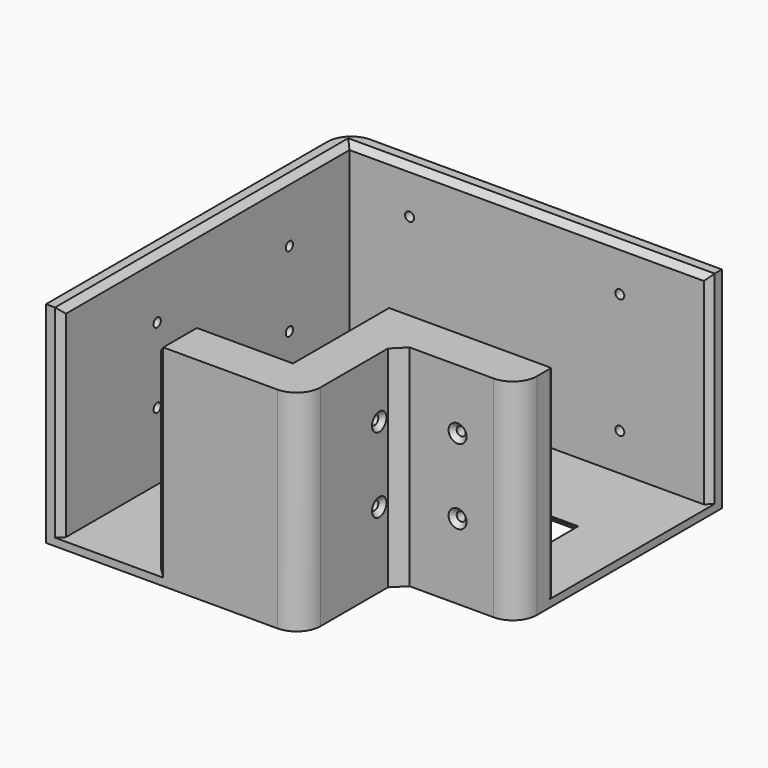
from build123d import *

# Parameters (mm, degrees)
F1_DEPTH        = 3.175
F2_DEPTH        = 88.9
F4_D            = 3.81
F4_DEPTH        = 25.4
F4_CSINK_D      = 7.62
F4_CSINK_ANGLE  = 90
F4_TIP          = 1.1446394792
F6_D            = 3.81
F6_DEPTH        = 25.4
F6_CSINK_D      = 7.62
F6_CSINK_ANGLE  = 90
F6_TIP          = 1.1446394792
F8_D            = 3.81
F8_DEPTH        = 25.4
F8_CSINK_D      = 7.62
F8_CSINK_ANGLE  = 90
F8_TIP          = 1.1446394792
F10_D           = 3.81
F10_DEPTH       = 25.4
F10_CSINK_D     = 7.62
F10_CSINK_ANGLE = 90
F10_TIP         = 1.1446394792
F11_T1_DEPTH    = 88.9
F11_T3_DEPTH    = 6.4524666085
F11_T5_DEPTH    = 6.4524666085
F11_T7_DEPTH    = 98.7891495789
F11_T9_DEPTH    = 115.0282991577
F11_T11_DEPTH   = 53.7041495789
F11_T13_DEPTH   = 63.8641495789
F11_T15_DEPTH   = 99.7882991577
F11_T17_DEPTH   = 48.9882991577
F11_T23_DEPTH   = 63.8641495789
F11_T27_DEPTH   = 53.7041495789
F12_R           = 10.16
F13_T1_DEPTH    = 91.44
F13_T3_DEPTH    = 52.2520747895
F13_T5_DEPTH    = 40.64
F13_T7_DEPTH    = 158.9320747894
F13_T9_DEPTH    = 158.9320747894
F13_T11_DEPTH   = 88.591569985
F13_T13_DEPTH   = 92.2570747894
F13_T15_DEPTH   = 49.9301865966
F13_T17_DEPTH   = 40.64
F13_T19_DEPTH   = 89.1181118071
F13_T25_DEPTH   = 47.1720747894
F13_T29_DEPTH   = 97.9720747894
F13_T36_DEPTH   = 95.6501865965
F13_T40_DEPTH   = 97.9720747894
F13_T47_DEPTH   = 47.1720747894
F13_T51_DEPTH   = 58.7841495789
F13_T58_DEPTH   = 158.9320747894
F13_S59_R       = 10.16
F13_T60_DEPTH   = 81
F13_T64_DEPTH   = 158.9320747894
F13_S66_R       = 10.16
F13_T67_DEPTH   = 81
F13_T73_DEPTH   = 56.462261386
F13_T77_DEPTH   = 47.1720747894
F13_T84_DEPTH   = 47.1720747894
F13_T88_DEPTH   = 95.6501865965


# Not quite as in the source:
# - a fillet or chamfer that OpenCascade refuses, or shapes differently, is made with other operations: its cross-section is extruded or revolved along the edge and cut away or added
# - a feature of the source that left no trace in its solid (it failed there, or was rolled back) is left out
# - a feature names something its author has since deleted; it is built from what else it names


with BuildPart() as f1:
    # F0 (on Top) → F1 (new body)
    with BuildSketch(Plane.XY):
        Polygon((-206.9763107598, 19.3472499192), (-359.3763107598, 19.3472499192), (-359.3763107598, -133.0527500808), (-321.2763107598, -133.0527500808), (-321.2763107598, -110.1927500808), (-321.2763107598, -18.7527500808), (-232.3763107598, -18.7527500808), (-232.1581989527, -18.7527500808), (-232.1581989527, -59.3927500808), (-206.9763107598, -59.3927500808), align=None)
    extrude(amount=F1_DEPTH)

    # F0 (on Top) → F2 (join)
    with BuildSketch(Plane.XY):
        Polygon((-206.9763107598, -82.2527500808), (-206.9763107598, -59.3927500808), (-232.1581989527, -59.3927500808), (-232.3763107598, -59.3927500808), (-280.6363107598, -59.3927500808), (-280.6363107598, -110.1927500808), (-321.2763107598, -110.1927500808), (-321.2763107598, -133.0527500808), (-257.7763107598, -133.0527500808), (-257.7763107598, -82.2527500808), align=None)
        Polygon((-359.3763107598, -133.0527500808), (-359.3763107598, 19.3472499192), (-206.9763107598, 19.3472499192), (-206.9763107598, 25.6972499192), (-365.7263107598, 25.6972499192), (-365.7263107598, -133.0527500808), align=None)
    extrude(amount=F2_DEPTH)

    # F4
    with Locations(Plane.XZ.offset(82.2527500808)):
        with Locations((-232.3763107598, 63.5), (-232.3763107598, 31.75)):
            CounterSinkHole(F4_D / 2, F4_CSINK_D / 2, depth=F4_DEPTH, counter_sink_angle=F4_CSINK_ANGLE)
            with Locations((0, 0, -(F4_DEPTH + F4_TIP / 2))):  # 118° drill point
                Cone(0, F4_D / 2, F4_TIP, mode=Mode.SUBTRACT)

    # F6
    with Locations(Plane.YZ.offset(-257.7763107598)):
        with Locations((-91.9047519565, 63.5), (-91.9047519565, 31.75)):
            CounterSinkHole(F6_D / 2, F6_CSINK_D / 2, depth=F6_DEPTH, counter_sink_angle=F6_CSINK_ANGLE)
            with Locations((0, 0, -(F6_DEPTH + F6_TIP / 2))):  # 118° drill point
                Cone(0, F6_D / 2, F6_TIP, mode=Mode.SUBTRACT)

    # F8
    with Locations(Plane(origin=(-365.7263107598, 0, 0), x_dir=(0, -1, 0), z_dir=(-1, 0, 0))):
        with Locations((12.4027500808, 63.5), (82.2527500808, 63.5), (82.2527500808, 31.75), (12.4027500808, 31.75)):
            CounterSinkHole(F8_D / 2, F8_CSINK_D / 2, depth=F8_DEPTH, counter_sink_angle=F8_CSINK_ANGLE)
            with Locations((0, 0, -(F8_DEPTH + F8_TIP / 2))):  # 118° drill point
                Cone(0, F8_D / 2, F8_TIP, mode=Mode.SUBTRACT)

    # F10
    with Locations(Plane(origin=(0, 25.6972499192, 0), x_dir=(-1, 0, 0), z_dir=(0, 1, 0))):
        with Locations((245.0763107598, 69.85), (245.0763107598, 19.05), (333.9763107598, 19.05), (333.9763107598, 69.85)):
            CounterSinkHole(F10_D / 2, F10_CSINK_D / 2, depth=F10_DEPTH, counter_sink_angle=F10_CSINK_ANGLE)
            with Locations((0, 0, -(F10_DEPTH + F10_TIP / 2))):  # 118° drill point
                Cone(0, F10_D / 2, F10_TIP, mode=Mode.SUBTRACT)

    # F11: chamfer of 5.08 on 10 edges, made by hand

    # F11_s2 → F11_t1 (join)
    with BuildSketch(Plane.XY):
        Polygon((-252.6963107598, -82.2527500808), (-257.7763107598, -87.3327500808), (-257.7763107598, -82.2527500808), align=None)
    extrude(amount=F11_T1_DEPTH)

    # F11_s4 → F11_t3 (cut)
    with BuildSketch(Plane(origin=(-96.6078535597, 96.6078535597, 96.6078535597), x_dir=(-0.7071067812, -0.7071067812, 0), z_dir=(-0.5773502692, 0.5773502692, 0.5773502692))):
        Polygon((301.5025963442, -15.6618580633), (305.0946987926, -9.4401541166), (308.686801241, -15.6618580633), align=None)
    extrude(amount=F11_T3_DEPTH, mode=Mode.SUBTRACT)

    # F11_s6 → F11_t5 (cut)
    with BuildSketch(Plane(origin=(-99.9945202263, 99.9945202263, 99.9945202263), x_dir=(-0.7071067812, -0.7071067812, 0), z_dir=(-0.5773502692, 0.5773502692, 0.5773502692))):
        Polygon((240.4368547209, -13.5879567477), (236.8447522725, -19.8096606944), (244.0289571693, -19.8096606944), align=None)
    extrude(amount=F11_T5_DEPTH, mode=Mode.SUBTRACT)

    # F11_s8 → F11_t7 (cut)
    with BuildSketch(Plane.XY.offset(3.175)):
        Polygon((-316.1963107598, -110.1927500808), (-321.2763107598, -115.2727500808), (-321.2763107598, -110.1927500808), align=None)
        Polygon((-316.1963107598, -133.0527500808), (-321.2763107598, -127.9727500808), (-321.2763107598, -133.0527500808), align=None)
        Polygon((-206.9763107598, -64.4727500808), (-212.0563107598, -59.3927500808), (-206.9763107598, -59.3927500808), align=None)
    extrude(amount=F11_T7_DEPTH, mode=Mode.SUBTRACT)

    # F11_s10 → F11_t9 (cut)
    with BuildSketch(Plane.XY.offset(-13.0641495789)):
        Polygon((-275.5563107598, -59.3927500808), (-280.6363107598, -64.4727500808), (-280.6363107598, -59.3927500808), align=None)
    extrude(amount=F11_T9_DEPTH, mode=Mode.SUBTRACT)

    # F11_s12 → F11_t11 (cut)
    with BuildSketch(Plane.YZ.offset(-334.3404603386)):
        Polygon((-115.2727500808, 88.9), (-110.1927500808, 83.82), (-110.1927500808, 88.9), align=None)
    extrude(amount=F11_T11_DEPTH, mode=Mode.SUBTRACT)

    # F11_s14 → F11_t13 (cut)
    with BuildSketch(Plane.XZ.offset(46.328600502)):
        Polygon((-275.5563107598, 88.9), (-280.6363107598, 83.82), (-280.6363107598, 88.9), align=None)
    extrude(amount=F11_T13_DEPTH, mode=Mode.SUBTRACT)

    # F11_s16 → F11_t15 (cut)
    with BuildSketch(Plane.YZ.offset(-293.7004603386)):
        Polygon((-64.4727500808, 88.9), (-59.3927500808, 83.82), (-59.3927500808, 88.9), align=None)
    extrude(amount=F11_T15_DEPTH, mode=Mode.SUBTRACT)

    # F11_s18 → F11_t17 (cut)
    with BuildSketch(Plane.XZ.offset(97.128600502)):
        Polygon((-316.1963107598, 88.9), (-321.2763107598, 83.82), (-321.2763107598, 88.9), align=None)
    extrude(amount=F11_T17_DEPTH, mode=Mode.SUBTRACT)


with BuildPart() as f11_tool21:
    # F11_s22 → F11_t23 (new body)
    with BuildSketch(Plane.XZ.offset(59.3927500808)):
        Polygon((-275.5563107598, 88.9), (-280.6363107598, 83.82), (-280.6363107598, 88.9), align=None)
    extrude(amount=F11_T23_DEPTH)

    split(bisect_by=Plane.XZ.offset(110.1927500808), keep=Keep.TOP)


with BuildPart() as f11_tool25:
    # F11_s26 → F11_t27 (new body)
    with BuildSketch(Plane.YZ.offset(-267.5721611809)):
        Polygon((-115.2727500808, 88.9), (-110.1927500808, 83.82), (-110.1927500808, 88.9), align=None)
    extrude(amount=-F11_T27_DEPTH)

    split(bisect_by=Plane.YZ.offset(-280.6363107598), keep=Keep.TOP)


with BuildPart() as f11_tool21_1:
    add(f11_tool21.part)

    # F11_t29: intersect F11_tool25
    add(f11_tool25.part, mode=Mode.INTERSECT)


with BuildPart() as f1_1:
    add(f1.part)

    # F11_t19: cut F11_tool21
    add(f11_tool21_1.part, mode=Mode.SUBTRACT)

    # F12
    f12_edges = [f1_1.edges().sort_by_distance(p)[0] for p in [
        (-257.776311, -133.05275, 44.45),
        (-206.976311, -82.25275, 44.45),
        (-365.726311, 25.69725, 44.45),
    ]]
    fillet(f12_edges, radius=F12_R)

    # F13: chamfer of 2.54 on 11 edges, made by hand

    # F13_s2 → F13_t1 (cut)
    with BuildSketch(Plane.XZ.offset(18.7527500808)):
        Polygon((-323.8163107598, 0), (-321.2763107598, 2.54), (-321.2763107598, 0), align=None)
    extrude(amount=F13_T1_DEPTH, mode=Mode.SUBTRACT)

    # F13_s4 → F13_t3 (cut)
    with BuildSketch(Plane.XZ.offset(57.9406752914)):
        Polygon((-278.0963107598, 0), (-280.6363107598, 2.54), (-280.6363107598, 0), align=None)
    extrude(amount=F13_T3_DEPTH, mode=Mode.SUBTRACT)

    # F13_s6 → F13_t5 (cut)
    with BuildSketch(Plane.YZ.offset(-321.2763107598)):
        Polygon((-112.7327500808, 0), (-110.1927500808, 2.54), (-110.1927500808, 0), align=None)
    extrude(amount=F13_T5_DEPTH, mode=Mode.SUBTRACT)

    # F13_s8 → F13_t7 (cut)
    with BuildSketch(Plane.YZ.offset(-359.3763107598)):
        Polygon((21.8872499192, 88.9), (19.3472499192, 86.36), (19.3472499192, 88.9), align=None)
    extrude(amount=F13_T7_DEPTH, mode=Mode.SUBTRACT)

    # F13_s10 → F13_t9 (cut)
    with BuildSketch(Plane.XZ.offset(-19.3472499192)):
        Polygon((-361.9163107598, 88.9), (-359.3763107598, 86.36), (-359.3763107598, 88.9), align=None)
    extrude(amount=F13_T9_DEPTH, mode=Mode.SUBTRACT)

    # F13_s12 → F13_t11 (cut)
    with BuildSketch(Plane.XY.offset(3.175)):
        Polygon((-206.9763107598, -65.5248525292), (-207.7202595356, -63.728801305), (-206.9763107598, -64.4727500808), align=None)
    extrude(amount=F13_T11_DEPTH, mode=Mode.SUBTRACT)

    # F13_s14 → F13_t13 (cut)
    with BuildSketch(Plane.XY.offset(3.175)):
        Polygon((-206.9763107598, 21.8872499192), (-209.5163107598, 19.3472499192), (-206.9763107598, 19.3472499192), align=None)
        Polygon((-361.9163107598, -133.0527500808), (-359.3763107598, -130.5127500808), (-359.3763107598, -133.0527500808), align=None)
    extrude(amount=F13_T13_DEPTH, mode=Mode.SUBTRACT)

    # F13_s16 → F13_t15 (cut)
    with BuildSketch(Plane.YZ.offset(-282.0883855492)):
        Polygon((-61.9327500808, 0), (-59.3927500808, 2.54), (-59.3927500808, 0), align=None)
    extrude(amount=F13_T15_DEPTH, mode=Mode.SUBTRACT)

    # F13_s18 → F13_t17 (cut)
    with BuildSketch(Plane.XZ.offset(18.7527500808)):
        Polygon((-229.6181989527, 0), (-232.1581989527, 2.54), (-232.1581989527, 0), align=None)
    extrude(amount=F13_T17_DEPTH, mode=Mode.SUBTRACT)

    # F13_s20 → F13_t19 (cut)
    with BuildSketch(Plane.YZ.offset(-321.2763107598)):
        Polygon((-16.2127500808, 0), (-18.7527500808, 2.54), (-18.7527500808, 0), align=None)
    extrude(amount=F13_T19_DEPTH, mode=Mode.SUBTRACT)


with BuildPart() as f13_tool23:
    # F13_s24 → F13_t25 (new body)
    with BuildSketch(Plane.YZ.offset(-280.6363107598)):
        Polygon((-112.7327500808, 0), (-110.1927500808, 2.54), (-110.1927500808, 0), align=None)
    extrude(amount=-F13_T25_DEPTH)

    split(bisect_by=Plane.YZ.offset(-321.2763107598), keep=Keep.BOTTOM)


with BuildPart() as f13_tool27:
    # F13_s28 → F13_t29 (new body)
    with BuildSketch(Plane.XZ.offset(116.7248248703)):
        Polygon((-323.8163107598, 0), (-321.2763107598, 2.54), (-321.2763107598, 0), align=None)
    extrude(amount=-F13_T29_DEPTH)

    split(bisect_by=Plane.XZ.offset(110.1927500808), keep=Keep.TOP)


with BuildPart() as f13_tool23_1:
    add(f13_tool23.part)

    # F13_t31: intersect F13_tool27
    add(f13_tool27.part, mode=Mode.INTERSECT)


with BuildPart() as f1_2:
    add(f1_1.part)

    # F13_t21: cut F13_tool23
    add(f13_tool23_1.part, mode=Mode.SUBTRACT)


with BuildPart() as f13_tool34:
    # F13_s35 → F13_t36 (new body)
    with BuildSketch(Plane.YZ.offset(-327.8083855492)):
        Polygon((-16.2127500808, 0), (-18.7527500808, 2.54), (-18.7527500808, 0), align=None)
    extrude(amount=F13_T36_DEPTH)

    split(bisect_by=Plane.YZ.offset(-321.2763107598), keep=Keep.BOTTOM)


with BuildPart() as f13_tool38:
    # F13_s39 → F13_t40 (new body)
    with BuildSketch(Plane.XZ.offset(110.1927500808)):
        Polygon((-323.8163107598, 0), (-321.2763107598, 2.54), (-321.2763107598, 0), align=None)
    extrude(amount=-F13_T40_DEPTH)

    split(bisect_by=Plane.XZ.offset(18.7527500808), keep=Keep.BOTTOM)


with BuildPart() as f13_tool34_1:
    add(f13_tool34.part)

    # F13_t42: intersect F13_tool38
    add(f13_tool38.part, mode=Mode.INTERSECT)


with BuildPart() as f1_3:
    add(f1_2.part)

    # F13_t32: cut F13_tool34
    add(f13_tool34_1.part, mode=Mode.SUBTRACT)


with BuildPart() as f13_tool45:
    # F13_s46 → F13_t47 (new body)
    with BuildSketch(Plane.YZ.offset(-274.1042359703)):
        Polygon((-112.7327500808, 0), (-110.1927500808, 2.54), (-110.1927500808, 0), align=None)
    extrude(amount=-F13_T47_DEPTH)

    split(bisect_by=Plane.YZ.offset(-280.6363107598), keep=Keep.TOP)


with BuildPart() as f13_tool49:
    # F13_s50 → F13_t51 (new body)
    with BuildSketch(Plane.XZ.offset(57.9406752914)):
        Polygon((-278.0963107598, 0), (-280.6363107598, 2.54), (-280.6363107598, 0), align=None)
    extrude(amount=F13_T51_DEPTH)

    split(bisect_by=Plane.XZ.offset(110.1927500808), keep=Keep.TOP)


with BuildPart() as f13_tool45_1:
    add(f13_tool45.part)

    # F13_t53: intersect F13_tool49
    add(f13_tool49.part, mode=Mode.INTERSECT)


with BuildPart() as f1_4:
    add(f1_3.part)

    # F13_t43: cut F13_tool45
    add(f13_tool45_1.part, mode=Mode.SUBTRACT)


with BuildPart() as f13_tool56:
    # F13_s57 → F13_t58 (new body)
    with BuildSketch(Plane.YZ.offset(-365.9083855492)):
        Polygon((21.8872499192, 88.9), (19.3472499192, 86.36), (19.3472499192, 88.9), align=None)
    extrude(amount=F13_T58_DEPTH)

    # F13_s59 → F13_t60 (intersect, symmetric)
    with BuildSketch(Plane.XY.offset(87.6)):
        with Locations((-355.5663107598, 15.5372499192)):
            Circle(F13_S59_R)
    extrude(amount=F13_T60_DEPTH, both=True, mode=Mode.INTERSECT)

    split(bisect_by=Plane.YZ.offset(-359.3763107598), keep=Keep.BOTTOM)


with BuildPart() as f13_tool62:
    # F13_s63 → F13_t64 (new body)
    with BuildSketch(Plane.XZ.offset(133.0527500808)):
        Polygon((-361.9163107598, 88.9), (-359.3763107598, 86.36), (-359.3763107598, 88.9), align=None)
    extrude(amount=-F13_T64_DEPTH)

    split(bisect_by=Plane.XZ.offset(-19.3472499192), keep=Keep.BOTTOM)

    # F13_s66 → F13_t67 (intersect, symmetric)
    with BuildSketch(Plane.XY.offset(87.6)):
        with Locations((-355.5663107598, 15.5372499192)):
            Circle(F13_S66_R)
    extrude(amount=F13_T67_DEPTH, both=True, mode=Mode.INTERSECT)


with BuildPart() as f13_tool56_1:
    add(f13_tool56.part)

    # F13_t68: intersect F13_tool62
    add(f13_tool62.part, mode=Mode.INTERSECT)


with BuildPart() as f1_5:
    add(f1_4.part)

    # F13_t54: cut F13_tool56
    add(f13_tool56_1.part, mode=Mode.SUBTRACT)


with BuildPart() as f13_tool71:
    # F13_s72 → F13_t73 (new body)
    with BuildSketch(Plane.YZ.offset(-225.6261241632)):
        Polygon((-61.9327500808, 0), (-59.3927500808, 2.54), (-59.3927500808, 0), align=None)
    extrude(amount=-F13_T73_DEPTH)

    split(bisect_by=Plane.YZ.offset(-232.1581989527), keep=Keep.TOP)


with BuildPart() as f13_tool75:
    # F13_s76 → F13_t77 (new body)
    with BuildSketch(Plane.XZ.offset(18.7527500808)):
        Polygon((-229.6181989527, 0), (-232.1581989527, 2.54), (-232.1581989527, 0), align=None)
    extrude(amount=F13_T77_DEPTH)

    split(bisect_by=Plane.XZ.offset(59.3927500808), keep=Keep.TOP)


with BuildPart() as f13_tool71_1:
    add(f13_tool71.part)

    # F13_t79: intersect F13_tool75
    add(f13_tool75.part, mode=Mode.INTERSECT)


with BuildPart() as f1_6:
    add(f1_5.part)

    # F13_t69: cut F13_tool71
    add(f13_tool71_1.part, mode=Mode.SUBTRACT)


with BuildPart() as f13_tool82:
    # F13_s83 → F13_t84 (new body)
    with BuildSketch(Plane.XZ.offset(12.2206752914)):
        Polygon((-229.6181989527, 0), (-232.1581989527, 2.54), (-232.1581989527, 0), align=None)
    extrude(amount=F13_T84_DEPTH)

    split(bisect_by=Plane.XZ.offset(18.7527500808), keep=Keep.BOTTOM)


with BuildPart() as f13_tool86:
    # F13_s87 → F13_t88 (new body)
    with BuildSketch(Plane.YZ.offset(-321.2763107598)):
        Polygon((-16.2127500808, 0), (-18.7527500808, 2.54), (-18.7527500808, 0), align=None)
    extrude(amount=F13_T88_DEPTH)

    split(bisect_by=Plane.YZ.offset(-232.1581989527), keep=Keep.TOP)


with BuildPart() as f13_tool82_1:
    add(f13_tool82.part)

    # F13_t90: intersect F13_tool86
    add(f13_tool86.part, mode=Mode.INTERSECT)


with BuildPart() as f1_7:
    add(f1_6.part)

    # F13_t80: cut F13_tool82
    add(f13_tool82_1.part, mode=Mode.SUBTRACT)


solid = f1_7.part
